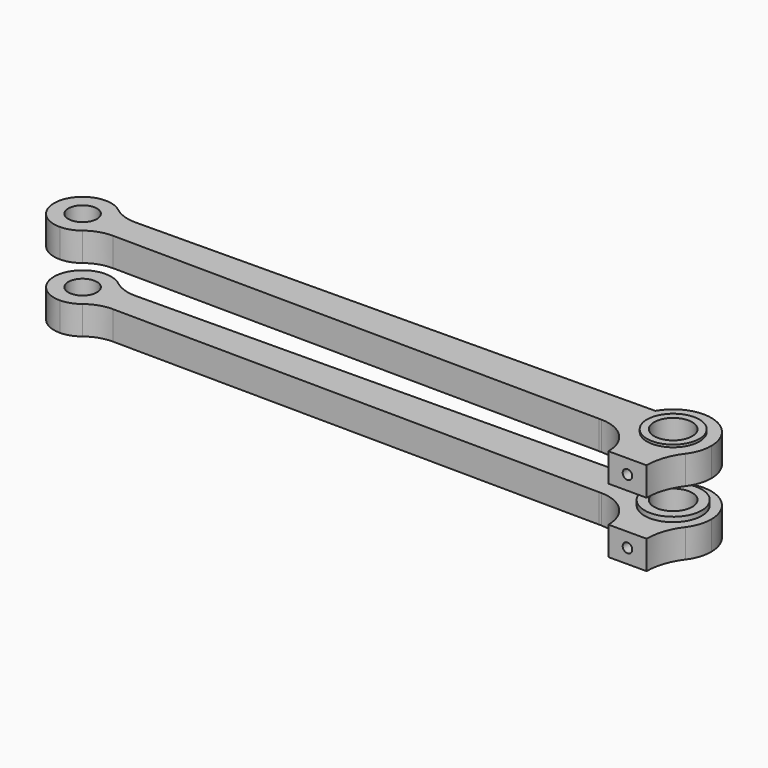
from build123d import *

# Parameters (mm, degrees)
F0_W      = 109.5375
F0_H      = 4.7625
F1_DEPTH  = 15.875
F3_DEPTH  = 4.7625
F4_R      = 2.38125
F5_DEPTH  = 4.7625
F6_R      = 4.7625
F7_DEPTH  = 0.79375
F8_R      = 4.365625
F9_DEPTH  = 0.396875
F10_R     = 3.175
F11_DEPTH = 6.35
F12_R     = 0.79375
F13_DEPTH = 3.175


# Not quite as in the source:
# - a length typed as a fraction of an inch, garbled in the dataset ("3 / 203.2 mm" for 3/8 in), is restored


with BuildPart() as f1:
    # F0 (on Front) → F1 (new body)
    with BuildSketch(Plane.XZ):
        with Locations((22.9201070249, 5.3867108949)):
            Rectangle(F0_W, F0_H)
    extrude(amount=F1_DEPTH)

    # F2 (on face) → F3 (cut)
    with BuildSketch(Plane(origin=(0, 0, 3.0054608949), x_dir=(1, 0, 0), z_dir=(0, 0, -1))):
        with BuildLine():
            ThreePointArc((67.1235889731, 1.6008932155), (66.4182398642, 2.3362702187), (65.8395957109, 3.175))
            Line((65.8395957109, 3.175), (62.9669316793, 3.2015159353))
            ThreePointArc((62.9669316793, 3.2015159353), (65.190207924, 2.7776190059), (67.1235889731, 1.6008932155))
        make_face()
        with BuildLine():
            Line((68.1638570249, 15.875), (-27.0861429751, 15.875))
            Line((-27.0861429751, 15.875), (-27.0861429751, 11.1125))
            ThreePointArc((-27.0861429751, 11.1125), (-25.5271603838, 10.8501088353), (-24.1399628876, 10.091848359))
            ThreePointArc((-24.1399628876, 10.091848359), (-22.262653003, 9.0713052051), (-20.1531120128, 8.73125))
            Line((-20.1531120128, 8.73125), (61.5207105875, 9.4851348166))
            Line((61.5207105875, 9.4851348166), (61.8725749266, 9.4883826771))
            ThreePointArc((61.8725749266, 9.4883826771), (66.3377291769, 11.3818749629), (68.1638570249, 15.875))
        make_face()
        with BuildLine():
            ThreePointArc((-24.1399628876, 2.608151641), (-25.5271603838, 1.8498911647), (-27.0861429751, 1.5875))
            Line((-27.0861429751, 1.5875), (-27.0861429751, 0))
            Line((-27.0861429751, 0), (71.3388570249, 0))
            ThreePointArc((71.3388570249, 0), (69.0843424521, 0.4136994651), (67.1235889731, 1.6008932155))
            ThreePointArc((67.1235889731, 1.6008932155), (65.190207924, 2.7776190059), (62.9669316793, 3.2015159353))
            Line((62.9669316793, 3.2015159353), (61.5207105875, 3.2148651834))
            Line((61.5207105875, 3.2148651834), (-20.1531120128, 3.96875))
            ThreePointArc((-20.1531120128, 3.96875), (-22.262653003, 3.6286947949), (-24.1399628876, 2.608151641))
        make_face()
        with BuildLine():
            Line((-27.0861429751, 11.1125), (-27.0861429751, 15.875))
            Line((-27.0861429751, 15.875), (-31.8486429751, 15.875))
            Line((-31.8486429751, 15.875), (-31.8486429751, 6.35))
            ThreePointArc((-31.8486429751, 6.35), (-30.4537390205, 9.7175960454), (-27.0861429751, 11.1125))
        make_face()
        with BuildLine():
            ThreePointArc((-27.0861429751, 1.5875), (-30.4537390205, 2.9824039546), (-31.8486429751, 6.35))
            Line((-31.8486429751, 6.35), (-31.8486429751, 0))
            Line((-31.8486429751, 0), (-27.0861429751, 0))
            Line((-27.0861429751, 0), (-27.0861429751, 1.5875))
        make_face()
        with BuildLine():
            Line((77.6888570249, 15.875), (74.5138570249, 15.875))
            ThreePointArc((74.5138570249, 15.875), (75.002648611, 12.8629305287), (76.4188570249, 10.16))
            ThreePointArc((76.4188570249, 10.16), (77.3629959675, 8.3580463142), (77.6888570249, 6.35))
            Line((77.6888570249, 6.35), (77.6888570249, 15.875))
        make_face()
        with BuildLine():
            ThreePointArc((77.6888570249, 6.35), (75.8289850854, 1.8598719395), (71.3388570249, 0))
            Line((71.3388570249, 0), (77.6888570249, 0))
            Line((77.6888570249, 0), (77.6888570249, 6.35))
        make_face()
    extrude(amount=-F3_DEPTH, mode=Mode.SUBTRACT)

    # F4 (on face) → F5 (cut)
    with BuildSketch(Plane(origin=(0, 0, 3.0054608949), x_dir=(1, 0, 0), z_dir=(0, 0, -1))):
        with Locations((-27.0861429751, 6.35)):
            Circle(F4_R)
    extrude(amount=-F5_DEPTH, mode=Mode.SUBTRACT)

    # F6 (on face) → F7 (join)
    with BuildSketch(Plane(origin=(0, 0, 3.0054608949), x_dir=(1, 0, 0), z_dir=(0, 0, -1))):
        with Locations((71.3388570249, 6.35)):
            Circle(F6_R)
    extrude(amount=F7_DEPTH)

    # F8 (on face) → F9 (join)
    with BuildSketch(Plane.XY.offset(7.7679608949)):
        with Locations((71.3388570249, -6.35)):
            Circle(F8_R)
    extrude(amount=F9_DEPTH)

    # F10 (on face) → F11 (cut)
    with BuildSketch(Plane(origin=(0, 0, 2.2117108949), x_dir=(1, 0, 0), z_dir=(0, 0, -1))):
        with Locations((71.3388570249, 6.35)):
            Circle(F10_R)
    extrude(amount=-F11_DEPTH, mode=Mode.SUBTRACT)

    # F12 (on face) → F13 (cut)
    with BuildSketch(Plane.XZ.offset(15.875)):
        with Locations((71.3388570249, 5.3867108949)):
            Circle(F12_R)
    extrude(amount=-F13_DEPTH, mode=Mode.SUBTRACT)


with BuildPart() as f15_1:
    # F15: instance of F1
    add(f1.part.mirror(Plane.XY))


solid = Compound([f1.part, f15_1.part])
